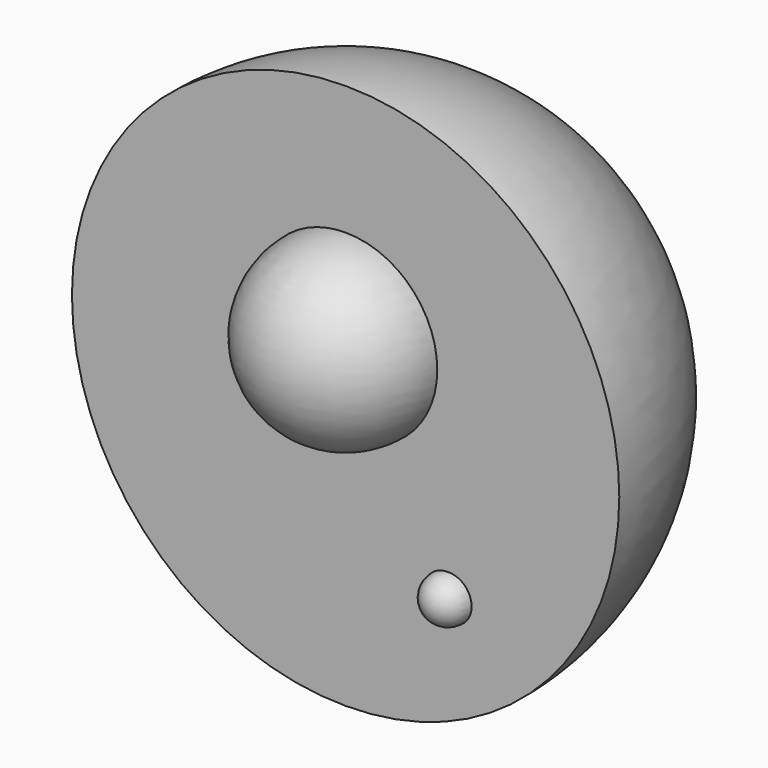
from build123d import *

# Parameters (mm, degrees)
F1_ANGLE = 180
F7_ANGLE = 180


# Not quite as in the source:
# - the program builds the solid bodies; features that only make, move or delete a surface that nothing else refers to are left out


with BuildPart() as f1:
    # F0 (on Front) → F1 (revolve)
    with BuildSketch(Plane.XZ):
        with BuildLine():
            Line((0, 60), (0, 0))
            ThreePointArc((0, 0), (30.0830305347, 30), (0, 60))
        make_face()
    revolve(axis=Axis((0, 0, 30), (0, 0, 1)), revolution_arc=F1_ANGLE)

    # F2 (on Front) → F3 (revolve)
    with BuildSketch(Plane.XZ):
        with BuildLine():
            Line((0, 45.8027541673), (0, 25.8027541673))
            ThreePointArc((0, 25.8027541673), (10.0749793548, 35.8027541673), (0, 45.8027541673))
        make_face()
    revolve(axis=Axis((0, 0, 35.8027541673), (0, 0, 1)))

    # F6 (on Front) → F7 (revolve)
    with BuildSketch(Plane.XZ):
        with BuildLine():
            ThreePointArc((11.2450128941, 11.6156497411), (13.8507385423, 14.1156497411), (11.2450128941, 16.6156497411))
            Line((11.2450128941, 16.6156497411), (11.2450128941, 11.6156497411))
        make_face()
    revolve(axis=Axis((11.2450128941, 0, 14.1156497411), (0, 0, -1)), revolution_arc=F7_ANGLE)


solid = f1.part
